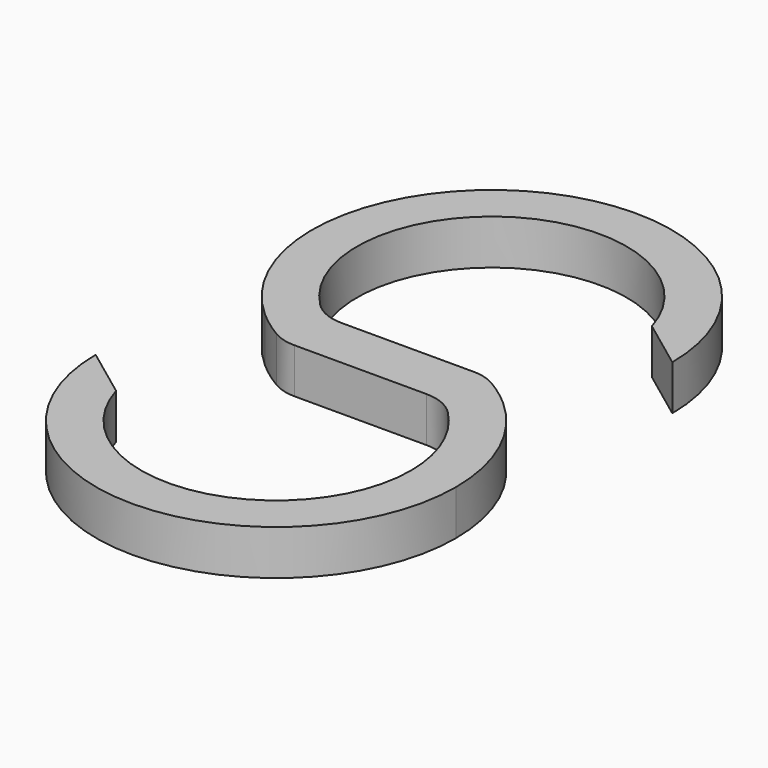
from build123d import *

# Parameters (mm, degrees)
F1_DEPTH    = 5
F2_T1_DEPTH = 31.594870106
F3_R        = 5


# Not quite as in the source:
# - a fillet or chamfer that OpenCascade refuses, or shapes differently, is made with other operations: its cross-section is extruded or revolved along the edge and cut away or added


with BuildPart() as f1:
    # F0 (on Top) → F1 (new body)
    with BuildSketch(Plane.XY):
        with BuildLine():
            ThreePointArc((20, 45), (-8.2287565553, 63.2287565553), (-13.2287565553, 30))
            ThreePointArc((-13.2287565553, 30), (-11.1540260033, 31.6008344344), (-8.8878037532, 32.9166666667))
            ThreePointArc((-8.8878037532, 32.9166666667), (-14.2521928137, 49.6770717335), (0, 60))
            ThreePointArc((0, 60), (10.6066017178, 55.6066017178), (15, 45))
            Line((15, 45), (20, 45))
        make_face()
        with BuildLine():
            ThreePointArc((-13.2287565553, 30), (-11.1540260033, 28.3991655656), (-8.8878037532, 27.0833333333))
            ThreePointArc((-8.8878037532, 27.0833333333), (-4.6770717335, 29.2521928137), (0, 30))
            ThreePointArc((0, 30), (-4.6770717335, 30.7478071863), (-8.8878037532, 32.9166666667))
            ThreePointArc((-8.8878037532, 32.9166666667), (-11.1540260033, 31.6008344344), (-13.2287565553, 30))
        make_face()
        with BuildLine():
            ThreePointArc((-8.8878037532, 32.9166666667), (-4.6770717335, 30.7478071863), (0, 30))
            Line((0, 30), (0, 32.9166666667))
            Line((0, 32.9166666667), (-8.8878037532, 32.9166666667))
        make_face()
        with BuildLine():
            ThreePointArc((0, 30), (-4.6770717335, 29.2521928137), (-8.8878037532, 27.0833333333))
            Line((-8.8878037532, 27.0833333333), (0, 27.0833333333))
            Line((0, 27.0833333333), (0, 30))
        make_face()
        with BuildLine():
            Line((0, 27.0833333333), (8.8878037532, 27.0833333333))
            ThreePointArc((8.8878037532, 27.0833333333), (4.6770717335, 29.2521928137), (0, 30))
            Line((0, 30), (0, 27.0833333333))
        make_face()
        with BuildLine():
            Line((0, 32.9166666667), (0, 30))
            ThreePointArc((0, 30), (4.6770717335, 30.7478071863), (8.8878037532, 32.9166666667))
            Line((8.8878037532, 32.9166666667), (0, 32.9166666667))
        make_face()
        with BuildLine():
            ThreePointArc((0, 30), (4.6770717335, 29.2521928137), (8.8878037532, 27.0833333333))
            ThreePointArc((8.8878037532, 27.0833333333), (11.1540260033, 28.3991655656), (13.2287565553, 30))
            ThreePointArc((13.2287565553, 30), (11.1540260033, 31.6008344344), (8.8878037532, 32.9166666667))
            ThreePointArc((8.8878037532, 32.9166666667), (4.6770717335, 30.7478071863), (0, 30))
        make_face()
        with BuildLine():
            ThreePointArc((15, 15), (10.6066017178, 4.3933982822), (0, 0))
            ThreePointArc((0, 0), (-10.6066017178, 4.3933982822), (-15, 15))
            Line((-15, 15), (-20, 15))
            ThreePointArc((-20, 15), (0, -5), (20, 15))
            ThreePointArc((20, 15), (18.2287565553, 23.2287565553), (13.2287565553, 30))
            ThreePointArc((13.2287565553, 30), (11.1540260033, 28.3991655656), (8.8878037532, 27.0833333333))
            ThreePointArc((8.8878037532, 27.0833333333), (13.3850113242, 21.7706330465), (15, 15))
        make_face()
    extrude(amount=F1_DEPTH)

    # F2: chamfer of 6 on 2 edges, made by hand

    # F2_s2 → F2_t1 (cut)
    with BuildSketch(Plane.XY.offset(-13.297435053)):
        with BuildLine():
            Line((-14.3747227125, 10.7142857143), (-20.1246117975, 15))
            Line((-20.1246117975, 15), (-15, 15))
            ThreePointArc((-15, 15), (-14.830161389, 12.7491527872), (-14.3747227125, 10.7142857143))
        make_face()
        with BuildLine():
            Line((20.1246117975, 45), (14.3747227125, 49.2857142857))
            ThreePointArc((14.3747227125, 49.2857142857), (14.830161389, 47.2508472128), (15, 45))
            Line((15, 45), (20.1246117975, 45))
        make_face()
    extrude(amount=F2_T1_DEPTH, mode=Mode.SUBTRACT)

    # F3
    f3_edges = [f1.edges().sort_by_distance(p)[0] for p in [
        (-8.887804, 32.916667, 2.5),
        (8.887804, 27.083333, 2.5),
        (8.887804, 32.916667, 2.5),
        (-8.887804, 27.083333, 2.5),
    ]]
    fillet(f3_edges, radius=F3_R)


solid = f1.part
